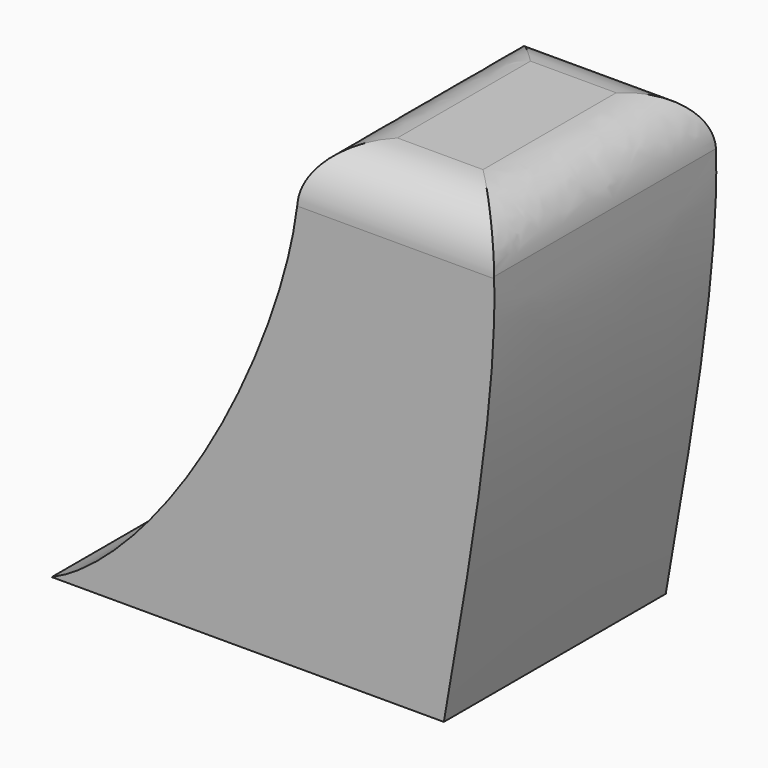
from build123d import *

# Parameters (mm, degrees)
F1_DEPTH = 25
F3_DEPTH = 52.7
F4_W     = 21.8509435654
F4_H     = 7.5018182397
F5_DEPTH = 59
F6_R     = 5


with BuildPart() as f1:
    # F0 (on Front) → F1 (new body)
    with BuildSketch(Plane.XZ):
        with BuildLine():
            add(Edge.make_bspline(
                [(40.403097868, 0), (44.3484185144, 22.4320712328), (51.8048986631, 64.8276858948), (2.8348392211, 27.1599391862), (0.8974329238, 8.5980973641), (0, 0)],
                knots=[0, 0, 0, 0, 0.3762323348, 0.7110623413, 1, 1, 1, 1], degree=3))
            Line((0, 0), (40.403097868, 0))
        make_face()
    extrude(amount=F1_DEPTH)

    # F2 (on Front) → F3 (cut)
    with BuildSketch(Plane.XZ):
        with BuildLine():
            add(Edge.make_bspline(
                [(0, 0), (4.1592267834, -2.743001842), (21.4151895882, 11.1218512251), (34.6891976083, 56.5742371109), (-4.672707747, 33.2384640146), (-4.8227010914, 3.1805618367), (0, 0)],
                knots=[0, 0, 0, 0, 0.222731211, 0.4925572792, 0.7417390034, 1, 1, 1, 1], degree=3))
        make_face()
    extrude(amount=F3_DEPTH, mode=Mode.SUBTRACT)

    # F4 (on Front) → F5 (cut)
    with BuildSketch(Plane.XZ):
        with Locations((36.8840396404, 45.3916192055)):
            Rectangle(F4_W, F4_H)
    extrude(amount=F5_DEPTH, mode=Mode.SUBTRACT)

    # F6
    f6_edges = [f1.edges().sort_by_distance(p)[0] for p in [
        (27.179604, -12.5, 41.64071),
        (35.804492, -25, 41.64071),
        (35.804492, 0, 41.64071),
        (44.42938, -12.5, 41.64071),
    ]]
    fillet(f6_edges, radius=F6_R)


solid = f1.part
